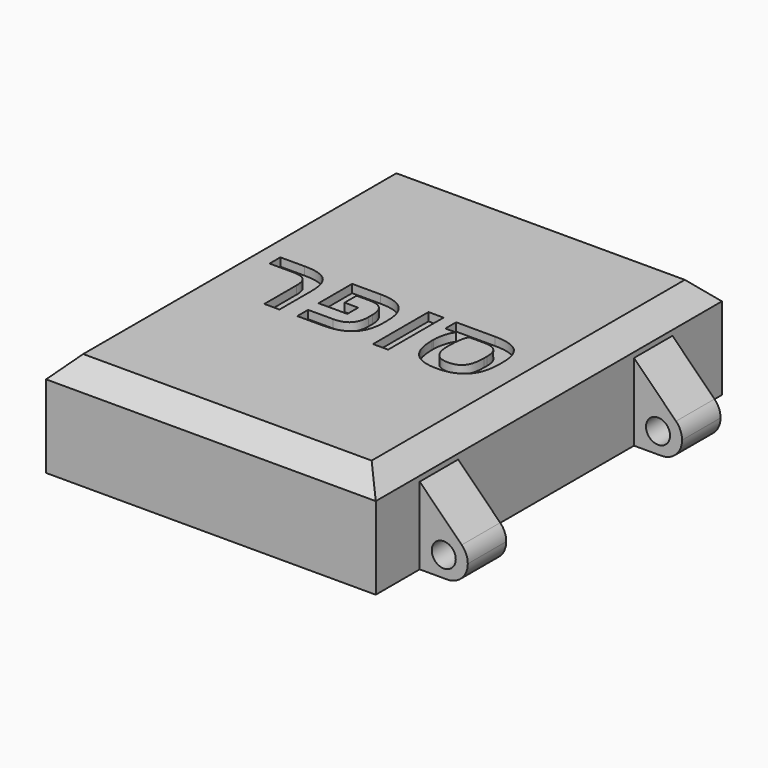
from build123d import *

# Parameters (mm, degrees)
F0_W          = 48
F0_H          = 63
F1_DEPTH      = 15
F2_W          = 44
F2_H          = 59
F3_DEPTH      = 13
F4_W          = 7
F4_H          = 7
F5_DEPTH      = 6
F6_R          = 1.75
F7_DEPTH      = 60.8
F8_R          = 2.99999
F9_W          = 44
F9_H          = 3
F10_DEPTH     = 13
F11_W         = 44
F11_H         = 8
F12_DEPTH     = 1
F13_W         = 2
F13_H         = 11
F13_H_2       = 10
F14_DEPTH     = 13
F15_SIZE      = 3
F16_SIZE      = 2
F18_DEPTH     = 7
F20_DEPTH     = 7
F21_TEXT_SIZE = 16.6666666667
F22_DEPTH     = 1.2


# Not quite as in the source:
# - a fillet or chamfer is up to 0.001 mm smaller than in the source, because OpenCascade refuses the exact size
# - Text() gives the source's letters only with a copy of the font that has no kerning and outlines rounded to 1/6400 em; it was checked with that copy


with BuildPart() as f1:
    # F0 (on Top) → F1 (new body)
    with BuildSketch(Plane.XY):
        with Locations((24, 31.5)):
            Rectangle(F0_W, F0_H)
    extrude(amount=F1_DEPTH)

    # F2 (on face) → F3 (cut)
    with BuildSketch(Plane(origin=(0, 0, 0), x_dir=(1, 0, 0), z_dir=(0, 0, -1))):
        with Locations((24, -31.5)):
            Rectangle(F2_W, F2_H)
    extrude(amount=-F3_DEPTH, mode=Mode.SUBTRACT)

    # F4 (on face) → F5 (join)
    with BuildSketch(Plane(origin=(0, 0, 0), x_dir=(1, 0, 0), z_dir=(0, 0, -1))):
        with Locations((51.5, -11.5)):
            Rectangle(F4_W, F4_H)
        with Locations((51.5, -50.5)):
            Rectangle(F4_W, F4_H)
    extrude(amount=-F5_DEPTH)

    # F6 (on face) → F7 (cut)
    with BuildSketch(Plane.XZ.offset(-8)):
        with Locations((51.5, 3)):
            Circle(F6_R)
    extrude(amount=-F7_DEPTH, mode=Mode.SUBTRACT)

    # F8 (radius 3 in the source; OpenCascade refuses exactly that, so slightly less here)
    f8_edges = [f1.edges().sort_by_distance(p)[0] for p in [
        (55, 11.5, 0),
        (55, 11.5, 6),
        (55, 50.5, 6),
        (55, 50.5, 0),
    ]]
    fillet(f8_edges, radius=F8_R)

    # F9 (on face) → F10 (join, through all)
    with BuildSketch(Plane(origin=(0, 0, 0), x_dir=(1, 0, 0), z_dir=(0, 0, -1))):
        with Locations((24, -33)):
            Rectangle(F9_W, F9_H)
    extrude(amount=-F10_DEPTH)

    # F11 (on face) → F12 (join)
    with BuildSketch(Plane(origin=(0, 0, 0), x_dir=(1, 0, 0), z_dir=(0, 0, -1))):
        with Locations((24, -38.5)):
            Rectangle(F11_W, F11_H)
        with Locations((24, -6)):
            Rectangle(F11_W, F11_H)
    extrude(amount=-F12_DEPTH)

    # F13 (on face) → F14 (join, through all)
    with BuildSketch(Plane(origin=(0, 0, 0), x_dir=(1, 0, 0), z_dir=(0, 0, -1))):
        with Locations((25, -37)):
            Rectangle(F13_W, F13_H)
        with Locations((25, -5)):
            Rectangle(F13_W, F13_H_2)
    extrude(amount=-F14_DEPTH)

    # F15
    f15_edges = [f1.edges().sort_by_distance(p)[0] for p in [
        (48, 31.5, 15),
        (24, 0, 15),
        (0, 31.5, 15),
        (24, 63, 15),
    ]]
    chamfer(f15_edges, length=F15_SIZE)

    # F16
    f16_edges = [f1.edges().sort_by_distance(p)[0] for p in [
        (24, 61, 13),
        (46, 47.75, 13),
        (46, 16.75, 13),
        (13, 2, 13),
        (36, 2, 13),
        (2, 16.75, 13),
        (2, 47.75, 13),
        (24, 31.5, 13),
        (13, 34.5, 13),
        (36, 34.5, 13),
    ]]
    chamfer(f16_edges, length=F16_SIZE)

    # F17 (on face) → F18 (join, through all)
    with BuildSketch(Plane.XZ.offset(-8)):
        with BuildLine():
            Line((48, 11.2426406871), (48, 6))
            Line((48, 6), (52, 6))
            ThreePointArc((52, 6), (53.1480502971, 5.7716385975), (54.1213203436, 5.1213203436))
            Line((54.1213203436, 5.1213203436), (48, 11.2426406871))
        make_face()
    extrude(amount=-F18_DEPTH)

    # F19 (on face) → F20 (join, through all)
    with BuildSketch(Plane.XZ.offset(-47)):
        with BuildLine():
            Line((48, 11.2426406871), (48, 6))
            Line((48, 6), (52, 6))
            ThreePointArc((52, 6), (53.1480502971, 5.7716385975), (54.1213203436, 5.1213203436))
            Line((54.1213203436, 5.1213203436), (48, 11.2426406871))
        make_face()
    extrude(amount=-F20_DEPTH)

    # F21 (on face) → F22 (cut)
    with BuildSketch(Plane.XY.offset(15)):
        with Locations((5.3138020833, 25.5)):
            Text('רפוס', F21_TEXT_SIZE, font='Arimo', font_style=FontStyle.BOLD, text_align=(TextAlign.LEFT, TextAlign.BOTTOM))
    extrude(amount=-F22_DEPTH, mode=Mode.SUBTRACT)


solid = f1.part
